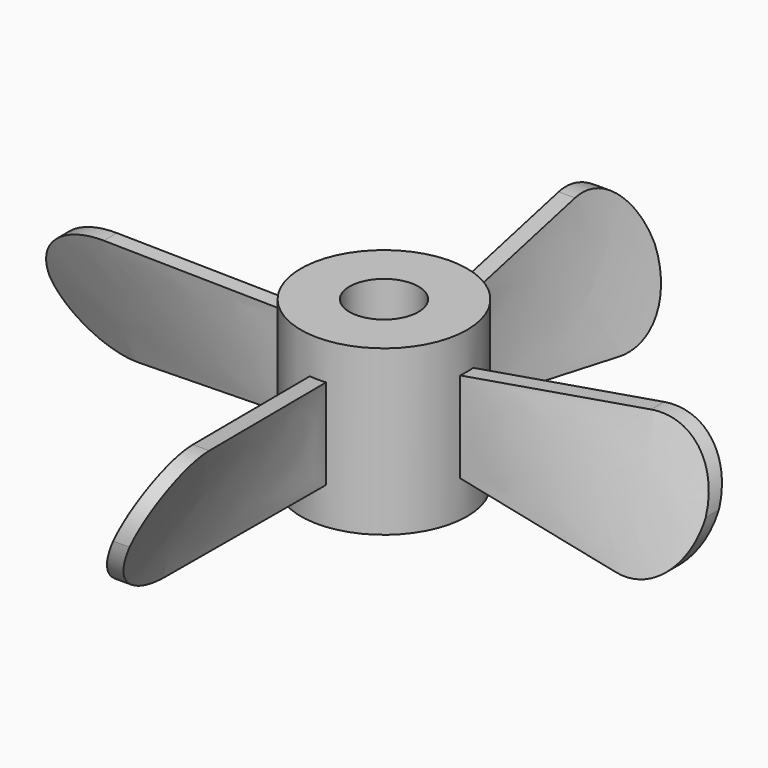
from build123d import *

# Parameters (mm, degrees)
F0_R          = 3.85802972
F2_DEPTH      = 3.81
F2_DEPTH_BACK = 3.81
F4_D          = 3.2004
F6_W          = 0.762
F6_H          = 4.191
F10_W         = 0.762
F10_H         = 4.191
F14_W         = 0.762
F14_H         = 4.191
F17_W         = 0.762
F17_H         = 4.191
F25_T1_DEPTH  = 17.6167754913
F25_T3_DEPTH  = 17.6167754913
F25_T5_DEPTH  = 17.6167754913
F25_T7_DEPTH  = 17.6167754913


# Not quite as in the source:
# - a fillet or chamfer that OpenCascade refuses, or shapes differently, is made with other operations: its cross-section is extruded or revolved along the edge and cut away or added


with BuildPart() as f2:
    # F0 (on Top) → F2 (new body, two sides)
    with BuildSketch(Plane.XY) as f2_sk:
        Circle(F0_R)
    extrude(amount=F2_DEPTH)
    extrude(f2_sk.sketch, amount=-F2_DEPTH_BACK)

    # F4 (through all)
    with Locations(Plane(origin=(0, 0, -3.81), x_dir=(1, 0, 0), z_dir=(0, 0, -1))):
        with Locations((0, 0)):
            Hole(F4_D / 2)

    # F6 (on offset) → F21 section 0
    with BuildSketch(Plane.YZ.offset(3.81)):
        Rectangle(F6_W, F6_H)
    # F20 (on offset) → F21 section 1
    with BuildSketch(Plane.YZ.offset(15.24)):
        Polygon((-1.8273555028, -3.2485676474), (-1.0653555028, -3.2485676474), (1.8273555028, 3.2485676474), (1.0653555028, 3.2485676474), align=None)
    loft()

    # F10 (on offset) → F22 section 0
    with BuildSketch(Plane.XZ.offset(-3.81)):
        Rectangle(F10_W, F10_H)
    # F11 (on offset) → F22 section 1
    with BuildSketch(Plane.XZ.offset(-15.24)):
        Polygon((-1.8273555028, 3.2485676474), (1.0653555028, -3.2485676474), (1.8273555028, -3.2485676474), (-1.0653555028, 3.2485676474), align=None)
    loft()

    # F14 (on offset) → F23 section 0
    with BuildSketch(Plane.YZ.offset(-3.81)):
        Rectangle(F14_W, F14_H)
    # F19 (on offset) → F23 section 1
    with BuildSketch(Plane.YZ.offset(-15.24)):
        Polygon((1.0653555028, -3.2485676474), (1.8273555028, -3.2485676474), (-1.0653555028, 3.2485676474), (-1.8273555028, 3.2485676474), align=None)
    loft()

    # F17 (on offset) → F24 section 0
    with BuildSketch(Plane.XZ.offset(3.81)):
        Rectangle(F17_W, F17_H)
    # F18 (on offset) → F24 section 1
    with BuildSketch(Plane.XZ.offset(15.24)):
        Polygon((-1.8273555028, -3.2485676474), (-1.0653555028, -3.2485676474), (1.8273555028, 3.2485676474), (1.0653555028, 3.2485676474), align=None)
    loft()

    # F25: fillet of radius 3.048 on 8 edges, made by hand

    # F25_s2 → F25_t1 (cut)
    with BuildSketch(Plane.XZ.offset(-7.3620322429)):
        with BuildLine():
            ThreePointArc((-11.8860680784, 2.9102202816), (-14.2362386728, 2.1384513865), (-15.24, -0.1223874509))
            Line((-15.24, -0.1223874509), (-15.24, 3.2485676474))
            Line((-15.24, 3.2485676474), (-11.8860680784, 2.9102202816))
        make_face()
        with BuildLine():
            ThreePointArc((11.8860680784, -2.9102202816), (14.2362386728, -2.1384513865), (15.24, 0.1223874509))
            Line((15.24, 0.1223874509), (15.24, -3.2485676474))
            Line((15.24, -3.2485676474), (11.8860680784, -2.9102202816))
        make_face()
    extrude(amount=F25_T1_DEPTH, mode=Mode.SUBTRACT)

    # F25_s4 → F25_t3 (cut)
    with BuildSketch(Plane.XZ.offset(-10.2547432484)):
        with BuildLine():
            ThreePointArc((-11.8860680784, -2.9102202816), (-14.2362386728, -2.1384513865), (-15.24, 0.1223874509))
            Line((-15.24, 0.1223874509), (-15.24, -3.2485676474))
            Line((-15.24, -3.2485676474), (-11.8860680784, -2.9102202816))
        make_face()
        with BuildLine():
            ThreePointArc((11.8860680784, 2.9102202816), (14.2362386728, 2.1384513865), (15.24, -0.1223874509))
            Line((15.24, -0.1223874509), (15.24, 3.2485676474))
            Line((15.24, 3.2485676474), (11.8860680784, 2.9102202816))
        make_face()
    extrude(amount=F25_T3_DEPTH, mode=Mode.SUBTRACT)

    # F25_s6 → F25_t5 (cut)
    with BuildSketch(Plane.YZ.offset(-7.3620322429)):
        with BuildLine():
            ThreePointArc((11.8860680784, -2.9102202816), (14.2362386728, -2.1384513865), (15.24, 0.1223874509))
            Line((15.24, 0.1223874509), (15.24, -3.2485676474))
            Line((15.24, -3.2485676474), (11.8860680784, -2.9102202816))
        make_face()
        with BuildLine():
            ThreePointArc((-11.8860680784, 2.9102202816), (-14.2362386728, 2.1384513865), (-15.24, -0.1223874509))
            Line((-15.24, -0.1223874509), (-15.24, 3.2485676474))
            Line((-15.24, 3.2485676474), (-11.8860680784, 2.9102202816))
        make_face()
    extrude(amount=F25_T5_DEPTH, mode=Mode.SUBTRACT)

    # F25_s8 → F25_t7 (cut)
    with BuildSketch(Plane.YZ.offset(-10.2547432484)):
        with BuildLine():
            ThreePointArc((11.8860680784, 2.9102202816), (14.2362386728, 2.1384513865), (15.24, -0.1223874509))
            Line((15.24, -0.1223874509), (15.24, 3.2485676474))
            Line((15.24, 3.2485676474), (11.8860680784, 2.9102202816))
        make_face()
        with BuildLine():
            ThreePointArc((-11.8860680784, -2.9102202816), (-14.2362386728, -2.1384513865), (-15.24, 0.1223874509))
            Line((-15.24, 0.1223874509), (-15.24, -3.2485676474))
            Line((-15.24, -3.2485676474), (-11.8860680784, -2.9102202816))
        make_face()
    extrude(amount=F25_T7_DEPTH, mode=Mode.SUBTRACT)


solid = f2.part
